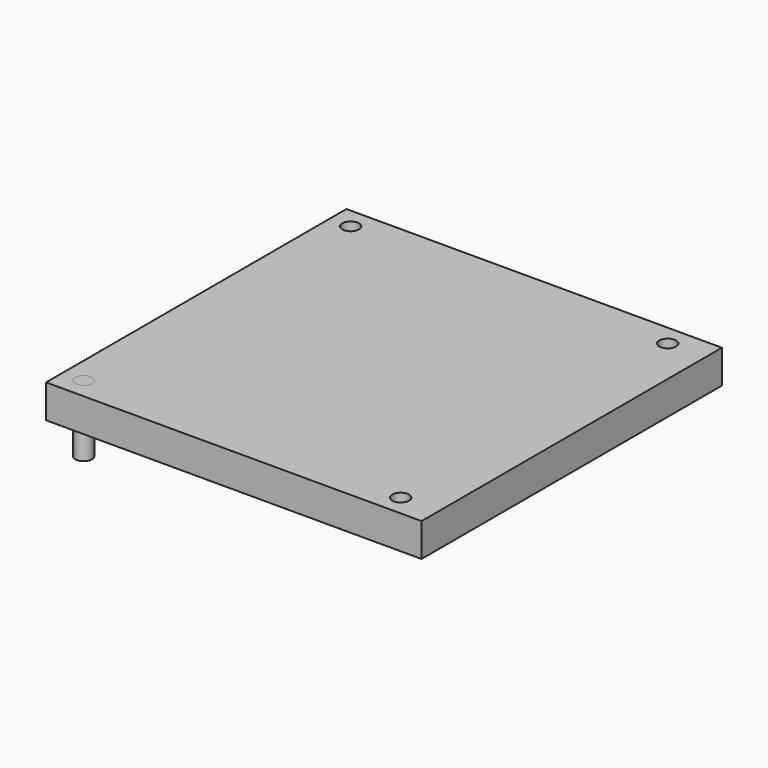
from build123d import *

# Parameters (mm, degrees)
F0_W     = 450
F0_H     = 450
F0_R     = 10
F1_DEPTH = 40
F2_R     = 10
F3_DEPTH = 80


# Not quite as in the source:
# - the program builds the solid bodies; features that only make, move or delete a surface that nothing else refers to are left out


with BuildPart() as f1:
    # F0 (on Top) → F1 (new body)
    with BuildSketch(Plane.XY):
        Rectangle(F0_W, F0_H)
        with Locations((-200, -200)):
            Circle(F0_R, mode=Mode.SUBTRACT)
        with Locations((180.0492778565, -200)):
            Circle(F0_R, mode=Mode.SUBTRACT)
        with Locations((-200, 200)):
            Circle(F0_R, mode=Mode.SUBTRACT)
        with Locations((180.0492778565, 200)):
            Circle(F0_R, mode=Mode.SUBTRACT)
    extrude(amount=F1_DEPTH)


with BuildPart() as f3:
    # F2 (on face) → F3 (new body)
    with BuildSketch(Plane.XY.offset(40)):
        with Locations((-200, -200)):
            Circle(F2_R)
    extrude(amount=-F3_DEPTH)


solid = Compound([f1.part, f3.part])
